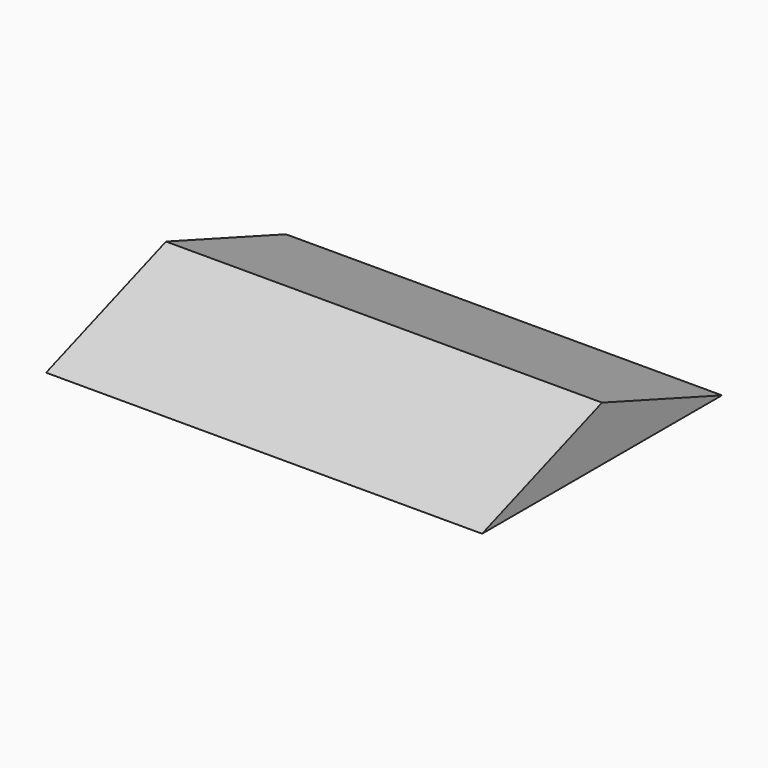
from build123d import *

# Parameters (mm, degrees)
F0_W       = 64
F0_H       = 44
F1_DEPTH   = 8
F2_SIZE2   = 21.99999
F2_SIZE    = 7.99999
F2_2_SIZE2 = 21.99999
F2_2_SIZE  = 7.99999


# Not quite as in the source:
# - a fillet or chamfer is up to 0.001 mm smaller than in the source, because OpenCascade refuses the exact size


with BuildPart() as f1:
    # F0 (on Top) → F1 (new body)
    with BuildSketch(Plane.XY):
        Rectangle(F0_W, F0_H)
    extrude(amount=F1_DEPTH)

    # F2 (size 8 and 22 in the source; OpenCascade refuses exactly that, so slightly less here)
    f2_edges = [f1.edges().sort_by_distance(p)[0] for p in [
        (0, -22, 8),
    ]]
    f2_side = f1.faces().sort_by_distance((0, -22, 4))[0]
    chamfer(f2_edges, length=F2_SIZE, length2=F2_SIZE2, reference=f2_side)

    # F2#2 (size 8 and 22 in the source; OpenCascade refuses exactly that, so slightly less here)
    f2_2_edges = [f1.edges().sort_by_distance(p)[0] for p in [
        (0, 22, 8),
    ]]
    f2_2_side = f1.faces().sort_by_distance((0, 22, 4))[0]
    chamfer(f2_2_edges, length=F2_2_SIZE, length2=F2_2_SIZE2, reference=f2_2_side)


solid = f1.part
